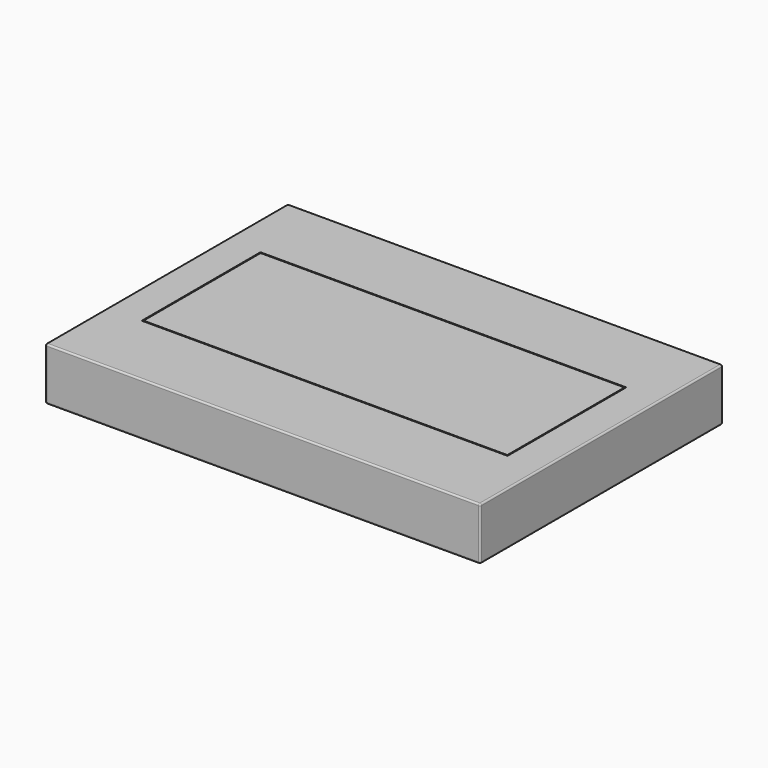
from build123d import *

# Parameters (mm, degrees)
F0_W     = 132
F0_H     = 92
F1_DEPTH = 16
F2_T     = -1
F3_R     = 0.49999
F4_W     = 111
F4_H     = 45
F5_DEPTH = 2
F6_W     = 110.3999990821
F6_H     = 44.3999990821
F7_DEPTH = 0.6


# Not quite as in the source:
# - a fillet or chamfer is up to 0.001 mm smaller than in the source, because OpenCascade refuses the exact size


with BuildPart() as f1:
    # F0 (on Top) → F1 (new body)
    with BuildSketch(Plane.XY):
        Rectangle(F0_W, F0_H)
    extrude(amount=F1_DEPTH)

    # F2
    f2_openings = [f1.faces().sort_by_distance(p)[0] for p in [
        (0, 0, 0),
    ]]
    offset(amount=F2_T, openings=f2_openings)

    # F3 (radius 0.5 in the source; OpenCascade refuses exactly that, so slightly less here)
    f3_edges = [f1.edges().sort_by_distance(p)[0] for p in [
        (66, -46, 8),
        (-66, -46, 8),
        (0, -46, 0),
        (0, -46, 16),
        (66, 46, 8),
        (66, 0, 16),
        (0, 46, 16),
        (-66, 0, 16),
        (-66, 46, 8),
        (0, 46, 0),
        (66, 0, 0),
        (-66, 0, 0),
        (0, -45, 0),
        (-65, -45, 7.5),
        (0, -45, 15),
        (65, -45, 7.5),
        (65, 0, 15),
        (0, 45, 15),
        (-65, 0, 15),
        (65, 45, 7.5),
        (0, 45, 0),
        (-65, 45, 7.5),
        (65, 0, 0),
        (-65, 0, 0),
    ]]
    fillet(f3_edges, radius=F3_R)

    # F4 (on face) → F5 (cut)
    with BuildSketch(Plane.XY.offset(16)):
        Rectangle(F4_W, F4_H)
    extrude(amount=-F5_DEPTH, mode=Mode.SUBTRACT)


with BuildPart() as f7:
    # F6 (on face) → F7 (new body)
    with BuildSketch(Plane.XY.offset(16)):
        Rectangle(F6_W, F6_H)
    extrude(amount=-F7_DEPTH)


solid = Compound([f1.part, f7.part])
